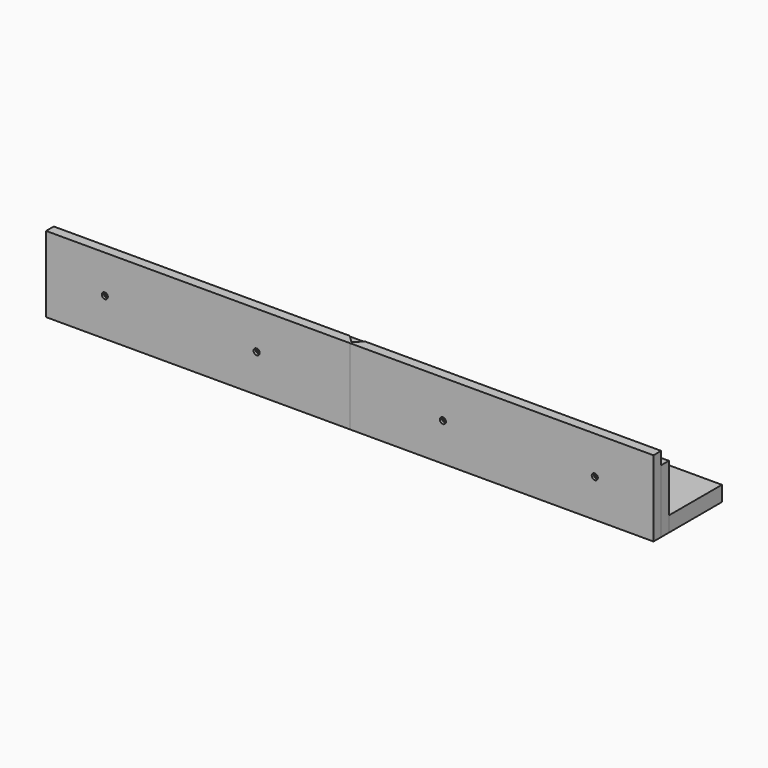
from build123d import *

# Parameters (mm, degrees)
F1_DEPTH  = 19
F3_DEPTH  = 30
F5_DEPTH  = 19
F7_W      = 19
F7_H      = 120.2081528017
F7_R      = 25
F8_DEPTH  = 19
F11_W     = 600
F11_H     = 25
F12_DEPTH = 19
F13_SIZE  = 15
F14_R     = 6
F14_R_2   = 3
F15_DEPTH = 5
F18_DEPTH = 108
F19_DEPTH = 108


# Not quite as in the source:
# - a feature names something its author has since deleted; it is built from what else it names


with BuildPart() as f1:
    # F0 (on Front) → F1 (new body)
    with BuildSketch(Plane.XZ):
        with BuildLine():
            Line((-600, 125), (-600, 0))
            Line((-600, 0), (-35, 0))
            Line((-35, 0), (-35, 35))
            ThreePointArc((-35, 35), (-32.0710678119, 42.0710678119), (-25, 45))
            Line((-25, 45), (25, 45))
            ThreePointArc((25, 45), (32.0710678119, 42.0710678119), (35, 35))
            Line((35, 35), (35, 0))
            Line((35, 0), (600, 0))
            Line((600, 0), (600, 125))
            Line((600, 125), (-600, 125))
        make_face()
        with BuildLine():
            ThreePointArc((-492, 75), (-491.1213203436, 77.1213203436), (-489, 78))
            Line((-489, 78), (-460, 78))
            ThreePointArc((-460, 78), (-457.8786796564, 77.1213203436), (-457, 75))
            ThreePointArc((-457, 75), (-457.8786796564, 72.8786796564), (-460, 72))
            Line((-460, 72), (-489, 72))
            ThreePointArc((-489, 72), (-491.1213203436, 72.8786796564), (-492, 75))
        make_face(mode=Mode.SUBTRACT)
        with BuildLine():
            ThreePointArc((-192, 75), (-191.1213203436, 77.1213203436), (-189, 78))
            Line((-189, 78), (-160, 78))
            ThreePointArc((-160, 78), (-157.8786796564, 77.1213203436), (-157, 75))
            ThreePointArc((-157, 75), (-157.8786796564, 72.8786796564), (-160, 72))
            Line((-160, 72), (-189, 72))
            ThreePointArc((-189, 72), (-191.1213203436, 72.8786796564), (-192, 75))
        make_face(mode=Mode.SUBTRACT)
        with BuildLine():
            ThreePointArc((160, 72), (157.8786796564, 72.8786796564), (157, 75))
            ThreePointArc((157, 75), (157.8786796564, 77.1213203436), (160, 78))
            Line((160, 78), (189, 78))
            ThreePointArc((189, 78), (191.1213203436, 77.1213203436), (192, 75))
            ThreePointArc((192, 75), (191.1213203436, 72.8786796564), (189, 72))
            Line((189, 72), (160, 72))
        make_face(mode=Mode.SUBTRACT)
        with BuildLine():
            ThreePointArc((460, 72), (457.8786796564, 72.8786796564), (457, 75))
            ThreePointArc((457, 75), (457.8786796564, 77.1213203436), (460, 78))
            Line((460, 78), (489, 78))
            ThreePointArc((489, 78), (491.1213203436, 77.1213203436), (492, 75))
            ThreePointArc((492, 75), (491.1213203436, 72.8786796564), (489, 72))
            Line((489, 72), (460, 72))
        make_face(mode=Mode.SUBTRACT)
    extrude(amount=-F1_DEPTH)


with BuildPart() as f3:
    # F2 (on Top) → F3 (new body)
    with BuildSketch(Plane.XY):
        with BuildLine():
            Line((-600, 150), (-600, 19))
            Line((-600, 19), (-35, 19))
            Line((-35, 19), (-35, 40))
            ThreePointArc((-35, 40), (-32.0710678119, 47.0710678119), (-25, 50))
            Line((-25, 50), (25, 50))
            ThreePointArc((25, 50), (32.0710678119, 47.0710678119), (35, 40))
            Line((35, 40), (35, 19))
            Line((35, 19), (600, 19))
            Line((600, 19), (600, 150))
            Line((600, 150), (-600, 150))
        make_face()
    extrude(amount=F3_DEPTH)


with BuildPart() as f5:
    # F4 (on face) → F5 (new body)
    with BuildSketch(Plane.YZ.offset(-35)):
        Polygon((104, 30), (19, 115), (19, 30), (40, 30), align=None)
    extrude(amount=-F5_DEPTH)


with BuildPart() as f6_1:
    # F6: instance of F5
    add(f5.part.mirror(Plane.YZ))


with BuildPart() as f8:
    # F7 (on face) → F8 (new body)
    with BuildSketch(Plane(origin=(0, 67, 67), x_dir=(-1, 0, 0), z_dir=(0, 0.7071067812, 0.7071067812))):
        Polygon((54, -52.3259018078), (54, 67.8822509939), (35, 67.8822509939), (35, 7.7781745931), (35, -13.4350288425), (35, -52.3259018078), align=None)
        with Locations((-44.5, 7.7781745931)):
            Rectangle(F7_W, F7_H)
        Polygon((35, 7.7781745931), (35, 67.8822509939), (-35, 67.8822509939), (-35, -52.3259018078), (35, -52.3259018078), (35, -13.4350288425), align=None)
        with Locations((0, 7.7781745931)):
            Circle(F7_R, mode=Mode.SUBTRACT)
    extrude(amount=F8_DEPTH)

    # F17 (on face) → F18 (cut, through all)
    with BuildSketch(Plane(origin=(-54, 0, 0), x_dir=(0, -1, 0), z_dir=(-1, 0, 0))):
        Polygon((-35.8700576851, 125), (-29, 125), (-32.4350288425, 128.4350288425), align=None)
    extrude(amount=-F18_DEPTH, mode=Mode.SUBTRACT)

    # F17 (on face) → F19 (join, through all)
    with BuildSketch(Plane(origin=(-54, 0, 0), x_dir=(0, -1, 0), z_dir=(-1, 0, 0))):
        Polygon((-130.8700576851, 30), (-104, 30), (-117.4350288425, 43.4350288425), align=None)
        Polygon((-19, 115), (-19, 125), (-29, 125), align=None)
    extrude(amount=-F19_DEPTH)


with BuildPart() as f9_1:
    # F9: copy of F6_1
    add(f6_1.part.moved(Location((300, 0, 0))))


with BuildPart() as f10_1:
    # F10: copy of F5
    add(f5.part.moved(Location((-300, 0, 0))))


with BuildPart() as f12:
    # F11 (on face) → F12 (new body)
    with BuildSketch(Plane.XZ):
        with BuildLine():
            Line((-600, 125), (-600, 0))
            Line((-600, 0), (-35, 0))
            Line((-35, 0), (-35, 35))
            ThreePointArc((-35, 35), (-32.0710678119, 42.0710678119), (-25, 45))
            Line((-25, 45), (0, 45))
            Line((0, 45), (0, 125))
            Line((0, 125), (-600, 125))
        make_face()
        with BuildLine():
            Line((-489, 78), (-484, 78))
            Line((-484, 78), (-460, 78))
            ThreePointArc((-460, 78), (-457, 75), (-460, 72))
            Line((-460, 72), (-484, 72))
            Line((-484, 72), (-489, 72))
            ThreePointArc((-489, 72), (-492, 75), (-489, 78))
        make_face(mode=Mode.SUBTRACT)
        with BuildLine():
            Line((-189, 78), (-184, 78))
            Line((-184, 78), (-160, 78))
            ThreePointArc((-160, 78), (-157, 75), (-160, 72))
            Line((-160, 72), (-184, 72))
            Line((-184, 72), (-189, 72))
            ThreePointArc((-189, 72), (-192, 75), (-189, 78))
        make_face(mode=Mode.SUBTRACT)
        with BuildLine():
            Line((-35, 35), (-35, 0))
            Line((-35, 0), (0, 0))
            Line((0, 0), (0, 45))
            Line((0, 45), (-25, 45))
            ThreePointArc((-25, 45), (-32.0710678119, 42.0710678119), (-35, 35))
        make_face()
        with Locations((-300, 137.5)):
            Rectangle(F11_W, F11_H)
        with BuildLine():
            ThreePointArc((-484, 78), (-481.8786796564, 77.1213203436), (-481, 75))
            ThreePointArc((-481, 75), (-481.8786796564, 72.8786796564), (-484, 72))
            Line((-484, 72), (-460, 72))
            ThreePointArc((-460, 72), (-457, 75), (-460, 78))
            Line((-460, 78), (-484, 78))
        make_face()
        with BuildLine():
            ThreePointArc((-484, 72), (-487, 75), (-484, 78))
            Line((-484, 78), (-489, 78))
            ThreePointArc((-489, 78), (-492, 75), (-489, 72))
            Line((-489, 72), (-484, 72))
        make_face()
        with BuildLine():
            ThreePointArc((-184, 78), (-181.8786796564, 77.1213203436), (-181, 75))
            ThreePointArc((-181, 75), (-181.8786796564, 72.8786796564), (-184, 72))
            Line((-184, 72), (-160, 72))
            ThreePointArc((-160, 72), (-157, 75), (-160, 78))
            Line((-160, 78), (-184, 78))
        make_face()
        with BuildLine():
            ThreePointArc((-184, 72), (-187, 75), (-184, 78))
            Line((-184, 78), (-189, 78))
            ThreePointArc((-189, 78), (-192, 75), (-189, 72))
            Line((-189, 72), (-184, 72))
        make_face()
    extrude(amount=F12_DEPTH)

    # F13
    f13_edges = [f12.edges().sort_by_distance(p)[0] for p in [
        (0, 0, 75),
    ]]
    chamfer(f13_edges, length=F13_SIZE)

    # F14 (on face) → F15 (cut)
    with BuildSketch(Plane.XZ.offset(19)):
        with Locations((-484, 75)):
            Circle(F14_R)
        with Locations((-484, 75)):
            Circle(F14_R_2, mode=Mode.SUBTRACT)
        with Locations((-184, 75)):
            Circle(F14_R)
        with Locations((-184, 75)):
            Circle(F14_R_2, mode=Mode.SUBTRACT)
    extrude(amount=-F15_DEPTH, mode=Mode.SUBTRACT)


with BuildPart() as f16_1:
    # F16: instance of F12
    add(f12.part.mirror(Plane.YZ))


solid = Compound([f1.part, f3.part, f5.part, f6_1.part, f8.part, f9_1.part, f10_1.part, f12.part, f16_1.part])
